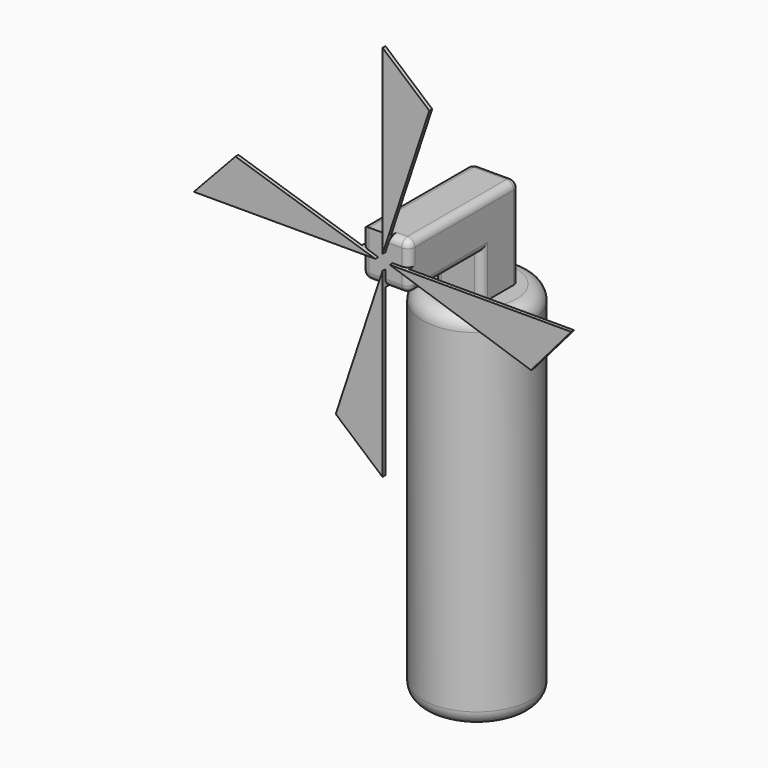
from build123d import *

# Parameters (mm, degrees)
F0_W           = 0.381
F0_H           = 2.54
F2_W           = 0.3302
F2_H           = 0.3302
F3_DEPTH       = 0.635
F4_W           = 0.3302
F4_H           = 0.3302
F5_DEPTH       = 0.635
F6_DEPTH       = 0.635
F8_DEPTH       = 0.0254
F9_DEPTH       = 0.0254
F11_DEPTH      = 0.0254
F13_DEPTH      = 0.0254
F15_DEPTH      = 0.0254
F16_T1_DEPTH   = 0.8636
F16_T3_DEPTH   = 0.5842
F16_T5_DEPTH   = 0.3048
F16_T7_DEPTH   = 0.5842
F16_T9_DEPTH   = 0.2286
F16_T11_DEPTH  = 1.0414
F16_T13_DEPTH  = 0.1181413534
F16_T15_DEPTH  = 0.1143
F16_T17_DEPTH  = 0.1143
F16_S21_W      = 0.051816
F16_S21_H      = 0.051816
F16_T22_DEPTH  = 0.051816
F16_S27_W      = 0.051816
F16_S27_H      = 0.051816
F16_T28_DEPTH  = 0.051816
F16_S33_W      = 0.051816
F16_S33_H      = 0.051816
F16_T34_DEPTH  = 0.051816
F16_S39_W      = 0.051816
F16_S39_H      = 0.051816
F16_T40_DEPTH  = 0.051816
F16_S45_W      = 0.051816
F16_S45_H      = 0.051816
F16_T46_DEPTH  = 0.051816
F16_T52_DEPTH  = 0.3787263164
F16_T57_DEPTH  = 0.3787263164
F16_T62_DEPTH  = 0.2451413534
F16_T67_DEPTH  = 0.2413
F16_T72_DEPTH  = 0.2043645658
F16_T77_DEPTH  = 0.2043645658
F16_T82_DEPTH  = 0.2413
F16_T87_DEPTH  = 0.2034354496
F16_T92_DEPTH  = 0.2034354496
F16_T97_DEPTH  = 0.2034354496
F16_T103_DEPTH = 0.4318
F16_T107_DEPTH = 0.7112
F16_T114_DEPTH = 0.4318
F16_T118_DEPTH = 0.7112
F17_R          = 0.1016


# Not quite as in the source:
# - a fillet or chamfer that OpenCascade refuses, or shapes differently, is made with other operations: its cross-section is extruded or revolved along the edge and cut away or added
# - a feature names something its author has since deleted; it is built from what else it names


with BuildPart() as f1:
    # F0 (on Front) → F1 (revolve)
    with BuildSketch(Plane.XZ):
        with Locations((0.1905, -0.0254572569)):
            Rectangle(F0_W, F0_H)
    revolve(axis=Axis((0, 0, -0.0254572569), (0, 0, -1)))

    # F2 (on face) → F3 (join)
    with BuildSketch(Plane.XY.offset(1.2445427431)):
        Rectangle(F2_W, F2_H)
    extrude(amount=F3_DEPTH)

    # F4 (on face) → F5 (join)
    with BuildSketch(Plane.XZ.offset(0.1651)):
        with Locations((0, 1.7144427431)):
            Rectangle(F4_W, F4_H)
    extrude(amount=F5_DEPTH)

    # F2 (on face) → F6 (join)
    with BuildSketch(Plane.XY.offset(1.2445427431)):
        Rectangle(F2_W, F2_H)
    extrude(amount=F6_DEPTH)

    # F7 (on face) → F8 (join)
    with BuildSketch(Plane.XZ.offset(0.8001)):
        Polygon((0, 3.0352427431), (0, 1.8795427431), (0.0378645504, 1.8795427431), (0.3274862888, 2.7538107431), align=None)
        Polygon((0, 1.8795427431), (0, 1.7652427431), (0.0378645504, 1.8795427431), align=None)
    extrude(amount=F8_DEPTH)

    # F7 (on face) → F9 (join)
    with BuildSketch(Plane.XZ.offset(0.8001)):
        Polygon((0, 3.0352427431), (0, 1.7652427431), (0.3274862888, 2.7538107431), align=None)
    extrude(amount=F9_DEPTH)

    # F10 (on face) → F11 (join)
    with BuildSketch(Plane.XZ.offset(0.8001)):
        Polygon((1.3208, 1.7144427431), (0.0508, 1.7144427431), (1.039368, 1.3869564543), align=None)
    extrude(amount=F11_DEPTH)

    # F12 (on face) → F13 (join)
    with BuildSketch(Plane.XZ.offset(0.8001)):
        Polygon((0, 0.3908380623), (0, 1.6608380623), (-0.3274862888, 0.6722700623), align=None)
    extrude(amount=F13_DEPTH)

    # F14 (on face) → F15 (join)
    with BuildSketch(Plane.XZ.offset(0.8001)):
        Polygon((-1.3206545556, 1.7182840966), (-0.0506545556, 1.7182840966), (-1.0291112121, 2.0306189544), align=None)
    extrude(amount=F15_DEPTH)

    # F16: fillet of radius 0.0508 on 16 edges, made by hand

    # F16_s2 → F16_t1 (cut)
    with BuildSketch(Plane.XZ.offset(-0.1143)):
        with BuildLine():
            ThreePointArc((0.1651, 1.8287427431), (0.1502210245, 1.8646637676), (0.1143, 1.8795427431))
            Line((0.1143, 1.8795427431), (0.1651, 1.8795427431))
            Line((0.1651, 1.8795427431), (0.1651, 1.8287427431))
        make_face()
    extrude(amount=F16_T1_DEPTH, mode=Mode.SUBTRACT)

    # F16_s4 → F16_t3 (cut)
    with BuildSketch(Plane.XZ.offset(0.1651)):
        with BuildLine():
            ThreePointArc((0.1651, 1.6001427431), (0.1502210245, 1.5642217186), (0.1143, 1.5493427431))
            Line((0.1143, 1.5493427431), (0.1651, 1.5493427431))
            Line((0.1651, 1.5493427431), (0.1651, 1.6001427431))
        make_face()
        with BuildLine():
            ThreePointArc((-0.1651, 1.6001427431), (-0.1502210245, 1.5642217186), (-0.1143, 1.5493427431))
            Line((-0.1143, 1.5493427431), (-0.1651, 1.5493427431))
            Line((-0.1651, 1.5493427431), (-0.1651, 1.6001427431))
        make_face()
    extrude(amount=F16_T3_DEPTH, mode=Mode.SUBTRACT)

    # F16_s6 → F16_t5 (cut)
    with BuildSketch(Plane.XY.offset(1.2445427431)):
        with BuildLine():
            ThreePointArc((0.1651, -0.1143), (0.1502210245, -0.1502210245), (0.1143, -0.1651))
            Line((0.1143, -0.1651), (0.1651, -0.1651))
            Line((0.1651, -0.1651), (0.1651, -0.1143))
        make_face()
        with BuildLine():
            ThreePointArc((-0.1143, -0.1651), (-0.1502210245, -0.1502210245), (-0.1651, -0.1143))
            Line((-0.1651, -0.1143), (-0.1651, -0.1651))
            Line((-0.1651, -0.1651), (-0.1143, -0.1651))
        make_face()
    extrude(amount=F16_T5_DEPTH, mode=Mode.SUBTRACT)

    # F16_s8 → F16_t7 (cut)
    with BuildSketch(Plane.XY.offset(1.2445427431)):
        with BuildLine():
            ThreePointArc((0.1651, 0.1143), (0.1502210245, 0.1502210245), (0.1143, 0.1651))
            Line((0.1143, 0.1651), (0.1651, 0.1651))
            Line((0.1651, 0.1651), (0.1651, 0.1143))
        make_face()
        with BuildLine():
            ThreePointArc((-0.1651, 0.1143), (-0.1502210245, 0.1502210245), (-0.1143, 0.1651))
            Line((-0.1143, 0.1651), (-0.1651, 0.1651))
            Line((-0.1651, 0.1651), (-0.1651, 0.1143))
        make_face()
    extrude(amount=F16_T7_DEPTH, mode=Mode.SUBTRACT)

    # F16_s10 → F16_t9 (cut)
    with BuildSketch(Plane.YZ.offset(-0.1143)):
        with BuildLine():
            ThreePointArc((0.1651, 1.8287427431), (0.1502210245, 1.8646637676), (0.1143, 1.8795427431))
            Line((0.1143, 1.8795427431), (0.1651, 1.8795427431))
            Line((0.1651, 1.8795427431), (0.1651, 1.8287427431))
        make_face()
    extrude(amount=F16_T9_DEPTH, mode=Mode.SUBTRACT)

    # F16_s12 → F16_t11 (cut)
    with BuildSketch(Plane.XZ.offset(-0.1143)):
        with BuildLine():
            ThreePointArc((-0.1651, 1.8287427431), (-0.1502210245, 1.8646637676), (-0.1143, 1.8795427431))
            Line((-0.1143, 1.8795427431), (-0.1651, 1.8795427431))
            Line((-0.1651, 1.8795427431), (-0.1651, 1.8287427431))
        make_face()
    extrude(amount=F16_T11_DEPTH, mode=Mode.SUBTRACT)

    # F16_s14 → F16_t13 (cut)
    with BuildSketch(Plane.XY.offset(1.6001427431)):
        with BuildLine():
            ThreePointArc((-0.1651, -0.7493), (-0.1502210245, -0.7852210245), (-0.1143, -0.8001))
            Line((-0.1143, -0.8001), (-0.1651, -0.8001))
            Line((-0.1651, -0.8001), (-0.1651, -0.7493))
        make_face()
    extrude(amount=F16_T13_DEPTH, mode=Mode.SUBTRACT)

    # F16_s16 → F16_t15 (cut)
    with BuildSketch(Plane.YZ):
        with BuildLine():
            ThreePointArc((-0.7493, 1.5493427431), (-0.7852210245, 1.5642217186), (-0.8001, 1.6001427431))
            Line((-0.8001, 1.6001427431), (-0.8001, 1.5493427431))
            Line((-0.8001, 1.5493427431), (-0.7493, 1.5493427431))
        make_face()
    extrude(amount=F16_T15_DEPTH, mode=Mode.SUBTRACT)

    # F16_s18 → F16_t17 (cut)
    with BuildSketch(Plane.XY.offset(1.7144427431)):
        with BuildLine():
            ThreePointArc((0.1651, -0.7493), (0.1502210245, -0.7852210245), (0.1143, -0.8001))
            Line((0.1143, -0.8001), (0.1651, -0.8001))
            Line((0.1651, -0.8001), (0.1651, -0.7493))
        make_face()
    extrude(amount=F16_T17_DEPTH, mode=Mode.SUBTRACT)


with BuildPart() as f16_tool20:
    # F16_s21 → F16_t22 (new body)
    with BuildSketch(Plane.XY.offset(1.8287427431)):
        with Locations((0.140208, 0.140208)):
            Rectangle(F16_S21_W, F16_S21_H)
    extrude(amount=F16_T22_DEPTH)

    # F16_s23 → F16_t24 (revolve, cut)
    with BuildSketch(Plane(origin=(0.1143, 0.1143, 1.8287427431), x_dir=(-0.7071067812, -0.7071067812, 0), z_dir=(-0.7071067812, 0.7071067812, 0))):
        with BuildLine():
            ThreePointArc((0, -0.0508), (0.0508, 0), (0, 0.0508))
            Line((0, 0.0508), (0, -0.0508))
        make_face()
    revolve(axis=Axis((0.1143, 0.1143, 1.8287427431), (0, 0, 1)), mode=Mode.SUBTRACT)


with BuildPart() as f1_1:
    add(f1.part)

    # F16_t19: cut F16_tool20
    add(f16_tool20.part, mode=Mode.SUBTRACT)


with BuildPart() as f16_tool26:
    # F16_s27 → F16_t28 (new body)
    with BuildSketch(Plane.XZ.offset(0.7493)):
        with Locations((0.140208, 1.8546507431)):
            Rectangle(F16_S27_W, F16_S27_H)
    extrude(amount=F16_T28_DEPTH)

    # F16_s29 → F16_t30 (revolve, cut)
    with BuildSketch(Plane(origin=(0.1143, -0.7493, 1.8287427431), x_dir=(-0.7071067812, 0, -0.7071067812), z_dir=(-0.7071067812, 0, 0.7071067812))):
        with BuildLine():
            ThreePointArc((0, -0.0508), (0.0508, 0), (0, 0.0508))
            Line((0, 0.0508), (0, -0.0508))
        make_face()
    revolve(axis=Axis((0.1143, -0.7493, 1.8287427431), (0, -1, 0)), mode=Mode.SUBTRACT)


with BuildPart() as f1_2:
    add(f1_1.part)

    # F16_t25: cut F16_tool26
    add(f16_tool26.part, mode=Mode.SUBTRACT)


with BuildPart() as f16_tool32:
    # F16_s33 → F16_t34 (new body)
    with BuildSketch(Plane.XZ.offset(0.7493)):
        with Locations((0.140208, 1.5742347431)):
            Rectangle(F16_S33_W, F16_S33_H)
    extrude(amount=F16_T34_DEPTH)

    # F16_s35 → F16_t36 (revolve, cut)
    with BuildSketch(Plane(origin=(0.1143, -0.7493, 1.6001427431), x_dir=(-0.7071067812, 0, 0.7071067812), z_dir=(0.7071067812, 0, 0.7071067812))):
        with BuildLine():
            ThreePointArc((0, -0.0508), (0.0508, 0), (0, 0.0508))
            Line((0, 0.0508), (0, -0.0508))
        make_face()
    revolve(axis=Axis((0.1143, -0.7493, 1.6001427431), (0, -1, 0)), mode=Mode.SUBTRACT)


with BuildPart() as f1_3:
    add(f1_2.part)

    # F16_t31: cut F16_tool32
    add(f16_tool32.part, mode=Mode.SUBTRACT)


with BuildPart() as f16_tool38:
    # F16_s39 → F16_t40 (new body)
    with BuildSketch(Plane.XY.offset(1.8287427431)):
        with Locations((-0.140208, 0.140208)):
            Rectangle(F16_S39_W, F16_S39_H)
    extrude(amount=F16_T40_DEPTH)

    # F16_s41 → F16_t42 (revolve, cut)
    with BuildSketch(Plane(origin=(-0.1143, 0.1143, 1.8287427431), x_dir=(0.7071067812, -0.7071067812, 0), z_dir=(-0.7071067812, -0.7071067812, 0))):
        with BuildLine():
            ThreePointArc((0, -0.0508), (0.0508, 0), (0, 0.0508))
            Line((0, 0.0508), (0, -0.0508))
        make_face()
    revolve(axis=Axis((-0.1143, 0.1143, 1.8287427431), (0, 0, 1)), mode=Mode.SUBTRACT)


with BuildPart() as f1_4:
    add(f1_3.part)

    # F16_t37: cut F16_tool38
    add(f16_tool38.part, mode=Mode.SUBTRACT)


with BuildPart() as f16_tool44:
    # F16_s45 → F16_t46 (new body)
    with BuildSketch(Plane.XZ.offset(0.7493)):
        with Locations((-0.140208, 1.5742347431)):
            Rectangle(F16_S45_W, F16_S45_H)
    extrude(amount=F16_T46_DEPTH)

    # F16_s47 → F16_t48 (revolve, cut)
    with BuildSketch(Plane(origin=(-0.1143, -0.7493, 1.6001427431), x_dir=(0.7071067812, 0, 0.7071067812), z_dir=(0.7071067812, 0, -0.7071067812))):
        with BuildLine():
            ThreePointArc((0, -0.0508), (0.0508, 0), (0, 0.0508))
            Line((0, 0.0508), (0, -0.0508))
        make_face()
    revolve(axis=Axis((-0.1143, -0.7493, 1.6001427431), (0, -1, 0)), mode=Mode.SUBTRACT)


with BuildPart() as f1_5:
    add(f1_4.part)

    # F16_t43: cut F16_tool44
    add(f16_tool44.part, mode=Mode.SUBTRACT)


with BuildPart() as f16_tool50:
    # F16_s51 → F16_t52 (new body)
    with BuildSketch(Plane.XY.offset(2.0065427431)):
        with BuildLine():
            ThreePointArc((-0.1651, -0.7493), (-0.1502210245, -0.7852210245), (-0.1143, -0.8001))
            Line((-0.1143, -0.8001), (-0.1651, -0.8001))
            Line((-0.1651, -0.8001), (-0.1651, -0.7493))
        make_face()
    extrude(amount=-F16_T52_DEPTH)

    split(bisect_by=Plane(origin=(0.493090904, 0, 1.5447141589), x_dir=(0, 1, 0), z_dir=(0.3040944775, 0, 0.9526418785)), keep=Keep.TOP)


with BuildPart() as f1_6:
    add(f1_5.part)

    # F16_t49: cut F16_tool50
    add(f16_tool50.part, mode=Mode.SUBTRACT)


with BuildPart() as f16_tool55:
    # F16_s56 → F16_t57 (new body)
    with BuildSketch(Plane.XY.offset(2.0065427431)):
        with BuildLine():
            ThreePointArc((-0.1651, -0.7493), (-0.1502210245, -0.7852210245), (-0.1143, -0.8001))
            Line((-0.1143, -0.8001), (-0.1651, -0.8001))
            Line((-0.1651, -0.8001), (-0.1651, -0.7493))
        make_face()
    extrude(amount=-F16_T57_DEPTH)

    split(bisect_by=Plane.XY.offset(1.7182840966), keep=Keep.BOTTOM)


with BuildPart() as f1_7:
    add(f1_6.part)

    # F16_t54: cut F16_tool55
    add(f16_tool55.part, mode=Mode.SUBTRACT)


with BuildPart() as f16_tool60:
    # F16_s61 → F16_t62 (new body)
    with BuildSketch(Plane.XY.offset(1.8452840966)):
        with BuildLine():
            ThreePointArc((-0.1651, -0.7493), (-0.1502210245, -0.7852210245), (-0.1143, -0.8001))
            Line((-0.1143, -0.8001), (-0.1651, -0.8001))
            Line((-0.1651, -0.8001), (-0.1651, -0.7493))
        make_face()
    extrude(amount=-F16_T62_DEPTH)

    split(bisect_by=Plane(origin=(0.493090904, 0, 1.5447141589), x_dir=(0, 1, 0), z_dir=(0.3040944775, 0, 0.9526418785)), keep=Keep.TOP)


with BuildPart() as f1_8:
    add(f1_7.part)

    # F16_t59: cut F16_tool60
    add(f16_tool60.part, mode=Mode.SUBTRACT)


with BuildPart() as f16_tool65:
    # F16_s66 → F16_t67 (new body)
    with BuildSketch(Plane.YZ.offset(-0.127)):
        with BuildLine():
            ThreePointArc((-0.7493, 1.5493427431), (-0.7852210245, 1.5642217186), (-0.8001, 1.6001427431))
            Line((-0.8001, 1.6001427431), (-0.8001, 1.5493427431))
            Line((-0.8001, 1.5493427431), (-0.7493, 1.5493427431))
        make_face()
    extrude(amount=F16_T67_DEPTH)

    split(bisect_by=Plane(origin=(-0.4957832071, 0, 0.1642397919), x_dir=(0, 1, 0), z_dir=(-0.9492682927, 0, 0.3144673409)), keep=Keep.TOP)


with BuildPart() as f1_9:
    add(f1_8.part)

    # F16_t64: cut F16_tool65
    add(f16_tool65.part, mode=Mode.SUBTRACT)


with BuildPart() as f16_tool70:
    # F16_s71 → F16_t72 (new body)
    with BuildSketch(Plane.YZ.offset(-0.1143)):
        with BuildLine():
            ThreePointArc((-0.7493, 1.5493427431), (-0.7852210245, 1.5642217186), (-0.8001, 1.6001427431))
            Line((-0.8001, 1.6001427431), (-0.8001, 1.5493427431))
            Line((-0.8001, 1.5493427431), (-0.7493, 1.5493427431))
        make_face()
    extrude(amount=F16_T72_DEPTH)

    split(bisect_by=Plane(origin=(-0.4957832071, 0, 0.1642397919), x_dir=(0, 1, 0), z_dir=(-0.9492682927, 0, 0.3144673409)), keep=Keep.TOP)


with BuildPart() as f1_10:
    add(f1_9.part)

    # F16_t69: cut F16_tool70
    add(f16_tool70.part, mode=Mode.SUBTRACT)


with BuildPart() as f16_tool75:
    # F16_s76 → F16_t77 (new body)
    with BuildSketch(Plane.YZ.offset(-0.1143)):
        with BuildLine():
            ThreePointArc((-0.7493, 1.5493427431), (-0.7852210245, 1.5642217186), (-0.8001, 1.6001427431))
            Line((-0.8001, 1.6001427431), (-0.8001, 1.5493427431))
            Line((-0.8001, 1.5493427431), (-0.7493, 1.5493427431))
        make_face()
    extrude(amount=F16_T77_DEPTH)

    split(bisect_by=Plane.YZ, keep=Keep.TOP)


with BuildPart() as f1_11:
    add(f1_10.part)

    # F16_t74: cut F16_tool75
    add(f16_tool75.part, mode=Mode.SUBTRACT)


with BuildPart() as f16_tool80:
    # F16_s81 → F16_t82 (new body)
    with BuildSketch(Plane.XY.offset(1.5874427431)):
        with BuildLine():
            ThreePointArc((0.1651, -0.7493), (0.1502210245, -0.7852210245), (0.1143, -0.8001))
            Line((0.1143, -0.8001), (0.1651, -0.8001))
            Line((0.1651, -0.8001), (0.1651, -0.7493))
        make_face()
    extrude(amount=F16_T82_DEPTH)

    split(bisect_by=Plane(origin=(0.5168085453, 0, 1.5600665049), x_dir=(0, 1, 0), z_dir=(-0.3144673409, 0, -0.9492682927)), keep=Keep.TOP)


with BuildPart() as f1_12:
    add(f1_11.part)

    # F16_t79: cut F16_tool80
    add(f16_tool80.part, mode=Mode.SUBTRACT)


with BuildPart() as f16_tool85:
    # F16_s86 → F16_t87 (new body)
    with BuildSketch(Plane.XY.offset(1.6001427431)):
        with BuildLine():
            ThreePointArc((0.1651, -0.7493), (0.1502210245, -0.7852210245), (0.1143, -0.8001))
            Line((0.1143, -0.8001), (0.1651, -0.8001))
            Line((0.1651, -0.8001), (0.1651, -0.7493))
        make_face()
    extrude(amount=F16_T87_DEPTH)

    split(bisect_by=Plane(origin=(0.5168085453, 0, 1.5600665049), x_dir=(0, 1, 0), z_dir=(-0.3144673409, 0, -0.9492682927)), keep=Keep.TOP)


with BuildPart() as f1_13:
    add(f1_12.part)

    # F16_t84: cut F16_tool85
    add(f16_tool85.part, mode=Mode.SUBTRACT)


with BuildPart() as f16_tool90:
    # F16_s91 → F16_t92 (new body)
    with BuildSketch(Plane.XY.offset(1.6001427431)):
        with BuildLine():
            ThreePointArc((0.1651, -0.7493), (0.1502210245, -0.7852210245), (0.1143, -0.8001))
            Line((0.1143, -0.8001), (0.1651, -0.8001))
            Line((0.1651, -0.8001), (0.1651, -0.7493))
        make_face()
    extrude(amount=F16_T92_DEPTH)

    split(bisect_by=Plane.XY.offset(1.7144427431), keep=Keep.TOP)


with BuildPart() as f1_14:
    add(f1_13.part)

    # F16_t89: cut F16_tool90
    add(f16_tool90.part, mode=Mode.SUBTRACT)


with BuildPart() as f16_tool95:
    # F16_s96 → F16_t97 (new body)
    with BuildSketch(Plane.YZ.offset(0.1143)):
        with BuildLine():
            ThreePointArc((-0.8001, 1.8287427431), (-0.7852210245, 1.8646637676), (-0.7493, 1.8795427431))
            Line((-0.7493, 1.8795427431), (-0.8001, 1.8795427431))
            Line((-0.8001, 1.8795427431), (-0.8001, 1.8287427431))
        make_face()
    extrude(amount=-F16_T97_DEPTH)

    split(bisect_by=Plane(origin=(-0.526949453, 0, 0.1745643403), x_dir=(0, 1, 0), z_dir=(0.9492682927, 0, -0.3144673409)), keep=Keep.TOP)


with BuildPart() as f1_15:
    add(f1_14.part)

    # F16_t94: cut F16_tool95
    add(f16_tool95.part, mode=Mode.SUBTRACT)


with BuildPart() as f16_tool101:
    # F16_s102 → F16_t103 (new body)
    with BuildSketch(Plane.XY.offset(1.2445427431)):
        with BuildLine():
            ThreePointArc((0.1651, -0.1143), (0.1502210245, -0.1502210245), (0.1143, -0.1651))
            Line((0.1143, -0.1651), (0.1651, -0.1651))
            Line((0.1651, -0.1651), (0.1651, -0.1143))
        make_face()
    extrude(amount=F16_T103_DEPTH)

    split(bisect_by=Plane.XY.offset(1.5493427431), keep=Keep.TOP)


with BuildPart() as f16_tool105:
    # F16_s106 → F16_t107 (new body)
    with BuildSketch(Plane.XZ.offset(0.0381)):
        with BuildLine():
            ThreePointArc((0.1651, 1.6001427431), (0.1502210245, 1.5642217186), (0.1143, 1.5493427431))
            Line((0.1143, 1.5493427431), (0.1651, 1.5493427431))
            Line((0.1651, 1.5493427431), (0.1651, 1.6001427431))
        make_face()
    extrude(amount=F16_T107_DEPTH)

    split(bisect_by=Plane.XZ.offset(0.1651), keep=Keep.BOTTOM)


with BuildPart() as f16_tool101_1:
    add(f16_tool101.part)

    # F16_t109: intersect F16_tool105
    add(f16_tool105.part, mode=Mode.INTERSECT)


with BuildPart() as f1_16:
    add(f1_15.part)

    # F16_t99: cut F16_tool101
    add(f16_tool101_1.part, mode=Mode.SUBTRACT)


with BuildPart() as f16_tool112:
    # F16_s113 → F16_t114 (new body)
    with BuildSketch(Plane.XY.offset(1.2445427431)):
        with BuildLine():
            ThreePointArc((-0.1143, -0.1651), (-0.1502210245, -0.1502210245), (-0.1651, -0.1143))
            Line((-0.1651, -0.1143), (-0.1651, -0.1651))
            Line((-0.1651, -0.1651), (-0.1143, -0.1651))
        make_face()
    extrude(amount=F16_T114_DEPTH)

    split(bisect_by=Plane.XY.offset(1.5493427431), keep=Keep.TOP)


with BuildPart() as f16_tool116:
    # F16_s117 → F16_t118 (new body)
    with BuildSketch(Plane.XZ.offset(0.0381)):
        with BuildLine():
            ThreePointArc((-0.1651, 1.6001427431), (-0.1502210245, 1.5642217186), (-0.1143, 1.5493427431))
            Line((-0.1143, 1.5493427431), (-0.1651, 1.5493427431))
            Line((-0.1651, 1.5493427431), (-0.1651, 1.6001427431))
        make_face()
    extrude(amount=F16_T118_DEPTH)

    split(bisect_by=Plane.XZ.offset(0.1651), keep=Keep.BOTTOM)


with BuildPart() as f16_tool112_1:
    add(f16_tool112.part)

    # F16_t120: intersect F16_tool116
    add(f16_tool116.part, mode=Mode.INTERSECT)


with BuildPart() as f1_17:
    add(f1_16.part)

    # F16_t110: cut F16_tool112
    add(f16_tool112_1.part, mode=Mode.SUBTRACT)

    # F17
    f17_edges = [f1_17.edges().sort_by_distance(p)[0] for p in [
        (-0.381, 0, 1.244543),
        (-0.381, 0, -1.295457),
    ]]
    fillet(f17_edges, radius=F17_R)


solid = f1_17.part
